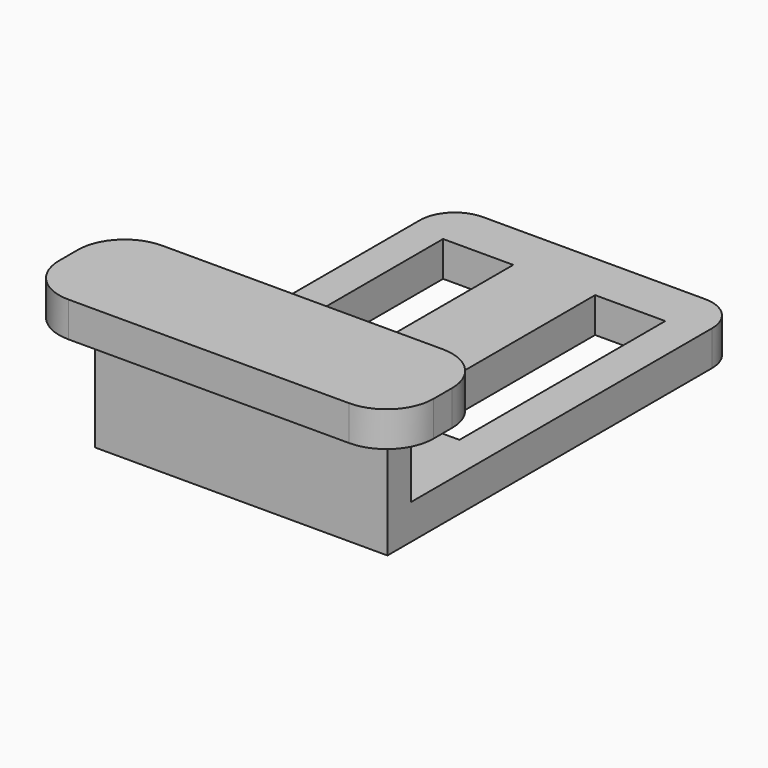
from build123d import *

# Parameters (mm, degrees)
F0_W     = 25
F0_H     = 3.598708484
F0_H_2   = 2.5
F0_H_3   = 31.6051654611
F0_W_2   = 6
F0_H_4   = 22
F1_DEPTH = 3
F2_DEPTH = 10
F3_START = 10
F3_DEPTH = 3
F4_R     = 4
F5_R     = 3


# Not quite as in the source:
# - a feature names something its author has since deleted; it is built from what else it names


with BuildPart() as f1:
    # F0 (on Top) → F1 (new body)
    with BuildSketch(Plane.XY):
        with Locations((0.1855289564, 2.9724632242)):
            Rectangle(F0_W, F0_H)
        with Locations((0.1855289564, -0.0768910178)):
            Rectangle(F0_W, F0_H_2)
        with Locations((0.1855289564, 20.5744001968)):
            Rectangle(F0_W, F0_H_3)
        with Locations((-6.4080492333, 21.2351317182)):
            Rectangle(F0_W_2, F0_H_4, mode=Mode.SUBTRACT)
        with Locations((6.5919507667, 21.2351317182)):
            Rectangle(F0_W_2, F0_H_4, mode=Mode.SUBTRACT)
    extrude(amount=F1_DEPTH)

    # F0 (on Top) → F2 (join)
    with BuildSketch(Plane.XY):
        with Locations((0.1855289564, -0.0768910178)):
            Rectangle(F0_W, F0_H_2)
    extrude(amount=F2_DEPTH)

    # F0 (on Top) → F3 (join)
    with BuildSketch(Plane.XY.offset(F3_START)):
        with Locations((0.1855289564, 2.9724632242)):
            Rectangle(F0_W, F0_H)
        Polygon((-12.3144710436, -1.3268910178), (-12.3144710436, 1.1731089822), (-12.3144710436, 4.7718174662), (-15.4697376937, 4.7718174662), (-15.4697376937, -5.2281825338), (16.5302623063, -5.2281825338), (16.5302623063, 4.7718174662), (12.6855289564, 4.7718174662), (12.6855289564, 1.1731089822), (12.6855289564, -1.3268910178), align=None)
        with Locations((0.1855289564, -0.0768910178)):
            Rectangle(F0_W, F0_H_2)
    extrude(amount=F3_DEPTH)

    # F4
    f4_edges = [f1.edges().sort_by_distance(p)[0] for p in [
        (16.530262, -5.228183, 11.5),
        (16.530262, 4.771817, 11.5),
        (-15.469738, -5.228183, 11.5),
        (-15.469738, 4.771817, 11.5),
    ]]
    fillet(f4_edges, radius=F4_R)

    # F5
    f5_edges = [f1.edges().sort_by_distance(p)[0] for p in [
        (-12.314471, 36.376983, 1.5),
        (12.685529, 36.376983, 1.5),
    ]]
    fillet(f5_edges, radius=F5_R)


solid = f1.part
